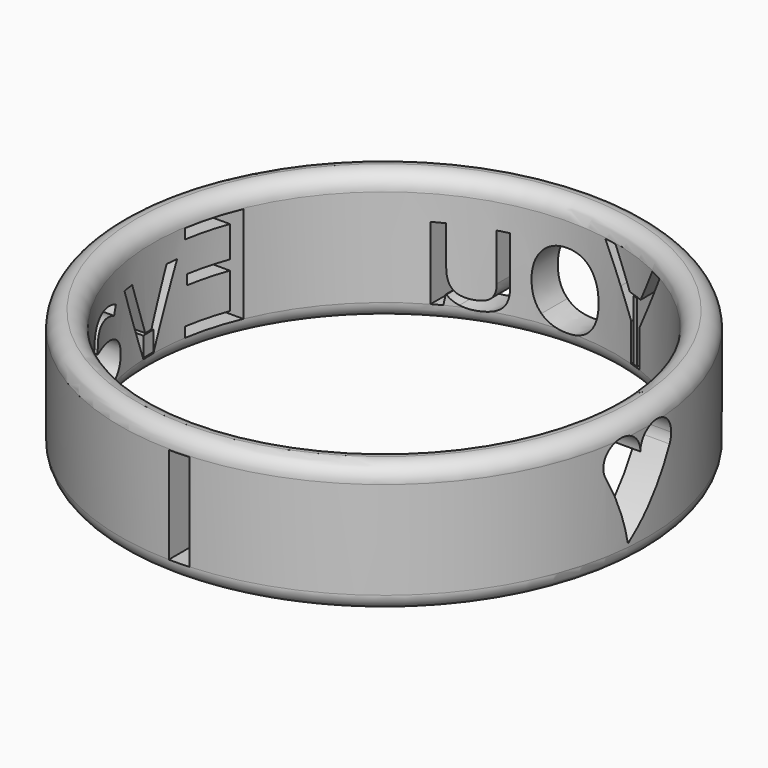
from build123d import *

# Parameters (mm, degrees)
F0_R          = 32.5
F0_R_2        = 28.5
F1_DEPTH      = 16
F3_TEXT_SIZE  = 16.6666666667
F4_DEPTH      = 25
F7_DEPTH      = 25
F15_TEXT_SIZE = 16.6666666667
F16_DEPTH     = 25
F17_DEPTH     = 25
F19_DEPTH     = 1.5
F19_TAPER     = -45
F21_DEPTH     = 2.7213541667
F22_DEPTH     = 0.15
F23_DEPTH     = 0.15
F24_DEPTH     = 7.6968030557
F25_DEPTH     = 0.15
F26_DEPTH     = 0.15
F24_FACE2_W   = 4.1758402468
F24_FACE2_H   = 7.3968030557
F27_DEPTH     = 0.4
F27_TAPER     = -45
F24_FACE3_W   = 4.2422939469
F24_FACE3_H   = 7.3968030557
F28_DEPTH     = 0.4
F28_TAPER     = -45


# Not quite as in the source:
# - a fillet or chamfer that OpenCascade refuses, or shapes differently, is made with other operations: its cross-section is extruded or revolved along the edge and cut away or added
# - Text() gives the source's letters only with a copy of the font that has no kerning and outlines rounded to 1/6400 em; it was checked with that copy


with BuildPart() as f1:
    # F0 (on Top) → F1 (new body)
    with BuildSketch(Plane.XY):
        Circle(F0_R)
        Circle(F0_R_2, mode=Mode.SUBTRACT)
    extrude(amount=F1_DEPTH)

    # F3 (on offset) → F4 (cut)
    with BuildSketch(Plane.XZ.offset(36)):
        with Locations((-2.0104166667, 2)):
            Text('I', F3_TEXT_SIZE, font='Open Sans', font_style=FontStyle.BOLD, text_align=(TextAlign.LEFT, TextAlign.BOTTOM))
    extrude(amount=-F4_DEPTH, mode=Mode.SUBTRACT)

    # F6 (on offset) → F7 (cut)
    with BuildSketch(Plane.YZ.offset(35.5)):
        with BuildLine():
            ThreePointArc((3.57761604, 10.5411187726), (0.7657574334, 9.2722506178), (-1.1375576102, 11.7))
            ThreePointArc((-1.1375576102, 11.7), (-3.0145179727, 9.2788800918), (-5.8270148983, 10.493237064))
            ThreePointArc((-5.8270148983, 10.493237064), (-4.0497196394, 6.5648465547), (-2.9116181205, 2.4060299726))
            ThreePointArc((-2.9116181205, 2.4060299726), (0.7233061967, 6.1622323434), (3.57761604, 10.5411187726))
        make_face()
        with BuildLine():
            ThreePointArc((-5.8270148983, 10.493237064), (-3.0145179727, 9.2788800918), (-1.1375576102, 11.7))
            ThreePointArc((-1.1375576102, 11.7), (-4.2605972477, 14.1211199082), (-5.8270148983, 10.493237064))
        make_face()
        with BuildLine():
            ThreePointArc((3.8624423898, 11.7), (1.3624423898, 14.2), (-1.1375576102, 11.7))
            ThreePointArc((-1.1375576102, 11.7), (0.7657574334, 9.2722506178), (3.57761604, 10.5411187726))
            ThreePointArc((3.57761604, 10.5411187726), (3.790191772, 11.1033150436), (3.8624423898, 11.7))
        make_face()
    extrude(amount=-F7_DEPTH, mode=Mode.SUBTRACT)

    # F15 (on line) → F16 (cut)
    with BuildSketch(Plane(origin=(-35.5, 0, 0), x_dir=(0, -1, 0), z_dir=(-1, 0, 0))):
        with Locations((-12.7682291667, 2)):
            Text('Eva', F15_TEXT_SIZE, font='Open Sans', text_align=(TextAlign.LEFT, TextAlign.BOTTOM))
        with BuildLine():
            add(Edge.make_bspline(
                [(7.4739583333, 3.3346354167), (7.9166666667, 2.953125), (8.7135416667, 2.953125)],
                knots=[0, 0, 0, 1, 1, 1], degree=2))
            add(Edge.make_bspline(
                [(8.7135416667, 2.953125), (9.9765625, 2.953125), (10.6966145833, 3.64453125)],
                knots=[0, 0, 0, 1, 1, 1], degree=2))
            add(Edge.make_bspline(
                [(10.6966145833, 3.64453125), (11.4166666667, 4.3359375), (11.4166666667, 5.5807291667)],
                knots=[0, 0, 0, 1, 1, 1], degree=2))
            Line((11.4166666667, 5.5807291667), (11.4166666667, 6.3854166667))
            Line((11.4166666667, 6.3854166667), (10.0651041667, 6.3307291667))
            add(Edge.make_bspline(
                [(10.0651041667, 6.3307291667), (8.453125, 6.2734375), (7.7421875, 5.8294270833)],
                knots=[0, 0, 0, 1, 1, 1], degree=2))
            add(Edge.make_bspline(
                [(7.7421875, 5.8294270833), (7.03125, 5.3854166667), (7.03125, 4.4505208333)],
                knots=[0, 0, 0, 1, 1, 1], degree=2))
            add(Edge.make_bspline(
                [(7.03125, 4.4505208333), (7.03125, 3.7161458333), (7.4739583333, 3.3346354167)],
                knots=[0, 0, 0, 1, 1, 1], degree=2))
        make_face()
    extrude(amount=-F16_DEPTH, mode=Mode.SUBTRACT)

    # F11 (on line) → F17 (cut)
    with BuildSketch(Plane(origin=(0, 35.5, 0), x_dir=(-1, 0, 0), z_dir=(0, 1, 0))):
        Polygon((-14.0989583333, 13.8984375), (-11.8328748379, 9.6968030557), (-10.3610019737, 9.6968030557), (-12.5859375, 13.8984375), align=None)
        Polygon((-10.3610019737, 9.6968030557), (-11.8328748379, 9.6968030557), (-10.1354166667, 6.5494791667), (-10.1354166667, 2), (-8.7369791667, 2), (-8.7369791667, 6.6145833333), (-7.0564696648, 9.6968030557), (-8.5026666772, 9.6968030557), (-9.4348958333, 7.9479166667), align=None)
        Polygon((-8.5026666772, 9.6968030557), (-10.3610019737, 9.6968030557), (-9.4348958333, 7.9479166667), align=None)
        Polygon((-6.2630208333, 13.8984375), (-8.5026666772, 9.6968030557), (-7.0564696648, 9.6968030557), (-4.765625, 13.8984375), align=None)
        with BuildLine():
            add(Edge.make_bspline(
                [(4.3645833333, 6.46875), (4.3645833333, 4.2864583333), (3.2669270833, 3.0611979167)],
                knots=[0, 0, 0, 1, 1, 1], degree=2))
            add(Edge.make_bspline(
                [(3.26171875, 9.8372395833), (4.3645833333, 8.5911458333), (4.3645833333, 6.46875)],
                knots=[0, 0, 0, 1, 1, 1], degree=2))
            add(Edge.make_bspline(
                [(0.2890625, 11.0833333333), (2.1588541667, 11.0833333333), (3.26171875, 9.8372395833)],
                knots=[0, 0, 0, 1, 1, 1], degree=2))
            add(Edge.make_bspline(
                [(-2.7395833333, 9.8658854167), (-1.6484375, 11.0833333333), (0.2890625, 11.0833333333)],
                knots=[0, 0, 0, 1, 1, 1], degree=2))
            add(Edge.make_bspline(
                [(-3.8307291667, 6.46875), (-3.8307291667, 8.6484375), (-2.7395833333, 9.8658854167)],
                knots=[0, 0, 0, 1, 1, 1], degree=2))
            add(Edge.make_bspline(
                [(-3.3255208333, 4.0104166667), (-3.8307291667, 5.0598958333), (-3.8307291667, 6.46875)],
                knots=[0, 0, 0, 1, 1, 1], degree=2))
            add(Edge.make_bspline(
                [(-1.8932291667, 2.3984375), (-2.8203125, 2.9609375), (-3.3255208333, 4.0104166667)],
                knots=[0, 0, 0, 1, 1, 1], degree=2))
            add(Edge.make_bspline(
                [(0.2317708333, 1.8359375), (-0.9661458333, 1.8359375), (-1.8932291667, 2.3984375)],
                knots=[0, 0, 0, 1, 1, 1], degree=2))
            add(Edge.make_bspline(
                [(3.2669270833, 3.0611979167), (2.1692708333, 1.8359375), (0.2317708333, 1.8359375)],
                knots=[0, 0, 0, 1, 1, 1], degree=2))
        make_face()
        with BuildLine():
            add(Edge.make_bspline(
                [(-2.4296875, 6.46875), (-2.4296875, 4.7578125), (-1.74609375, 3.86328125)],
                knots=[0, 0, 0, 1, 1, 1], degree=2))
            add(Edge.make_bspline(
                [(-1.75390625, 9.0638020833), (-2.4296875, 8.1927083333), (-2.4296875, 6.46875)],
                knots=[0, 0, 0, 1, 1, 1], degree=2))
            add(Edge.make_bspline(
                [(0.2473958333, 9.9348958333), (-1.078125, 9.9348958333), (-1.75390625, 9.0638020833)],
                knots=[0, 0, 0, 1, 1, 1], degree=2))
            add(Edge.make_bspline(
                [(2.2786458333, 9.0520833333), (1.5911458333, 9.9348958333), (0.2473958333, 9.9348958333)],
                knots=[0, 0, 0, 1, 1, 1], degree=2))
            add(Edge.make_bspline(
                [(2.9661458333, 6.46875), (2.9661458333, 8.1692708333), (2.2786458333, 9.0520833333)],
                knots=[0, 0, 0, 1, 1, 1], degree=2))
            add(Edge.make_bspline(
                [(2.2786458333, 3.859375), (2.9661458333, 4.75), (2.9661458333, 6.46875)],
                knots=[0, 0, 0, 1, 1, 1], degree=2))
            add(Edge.make_bspline(
                [(0.2630208333, 2.96875), (1.5911458333, 2.96875), (2.2786458333, 3.859375)],
                knots=[0, 0, 0, 1, 1, 1], degree=2))
            add(Edge.make_bspline(
                [(-1.74609375, 3.86328125), (-1.0625, 2.96875), (0.2630208333, 2.96875)],
                knots=[0, 0, 0, 1, 1, 1], degree=2))
        make_face(mode=Mode.SUBTRACT)
        with BuildLine():
            Line((8.0052083333, 5.1328125), (8.0052083333, 10.9192708333))
            Line((8.0052083333, 10.9192708333), (6.6380208333, 10.9192708333))
            Line((6.6380208333, 10.9192708333), (6.6380208333, 5.0833333333))
            add(Edge.make_bspline(
                [(7.4466145833, 2.609375), (6.6380208333, 3.3828125), (6.6380208333, 5.0833333333)],
                knots=[0, 0, 0, 1, 1, 1], degree=2))
            add(Edge.make_bspline(
                [(9.8828125, 1.8359375), (8.2552083333, 1.8359375), (7.4466145833, 2.609375)],
                knots=[0, 0, 0, 1, 1, 1], degree=2))
            add(Edge.make_bspline(
                [(11.5651041667, 2.1861979167), (10.828125, 1.8359375), (9.8828125, 1.8359375)],
                knots=[0, 0, 0, 1, 1, 1], degree=2))
            add(Edge.make_bspline(
                [(12.7161458333, 3.1953125), (12.3020833333, 2.5364583333), (11.5651041667, 2.1861979167)],
                knots=[0, 0, 0, 1, 1, 1], degree=2))
            Line((12.7161458333, 3.1953125), (12.7890625, 3.1953125))
            Line((12.7890625, 3.1953125), (12.984375, 2))
            Line((12.984375, 2), (14.0989583333, 2))
            Line((14.0989583333, 2), (14.0989583333, 10.9192708333))
            Line((14.0989583333, 10.9192708333), (12.7473958333, 10.9192708333))
            Line((12.7473958333, 10.9192708333), (12.7473958333, 6.2317708333))
            add(Edge.make_bspline(
                [(12.1015625, 3.7330729167), (12.7473958333, 4.4973958333), (12.7473958333, 6.2317708333)],
                knots=[0, 0, 0, 1, 1, 1], degree=2))
            add(Edge.make_bspline(
                [(10.0546875, 2.96875), (11.4557291667, 2.96875), (12.1015625, 3.7330729167)],
                knots=[0, 0, 0, 1, 1, 1], degree=2))
            add(Edge.make_bspline(
                [(8.5013020833, 3.5052083333), (8.9973958333, 2.96875), (10.0546875, 2.96875)],
                knots=[0, 0, 0, 1, 1, 1], degree=2))
            add(Edge.make_bspline(
                [(8.0052083333, 5.1328125), (8.0052083333, 4.0416666667), (8.5013020833, 3.5052083333)],
                knots=[0, 0, 0, 1, 1, 1], degree=2))
        make_face()
        with BuildLine():
            add(Edge.make_bspline(
                [(-1.75390625, 9.0638020833), (-2.4296875, 8.1927083333), (-2.4296875, 6.46875)],
                knots=[0, 0, 0, 1, 1, 1], degree=2))
            add(Edge.make_bspline(
                [(-2.4296875, 6.46875), (-2.4296875, 4.7578125), (-1.74609375, 3.86328125)],
                knots=[0, 0, 0, 1, 1, 1], degree=2))
            add(Edge.make_bspline(
                [(-1.74609375, 3.86328125), (-1.0625, 2.96875), (0.2630208333, 2.96875)],
                knots=[0, 0, 0, 1, 1, 1], degree=2))
            add(Edge.make_bspline(
                [(0.2630208333, 2.96875), (1.5911458333, 2.96875), (2.2786458333, 3.859375)],
                knots=[0, 0, 0, 1, 1, 1], degree=2))
            add(Edge.make_bspline(
                [(2.2786458333, 3.859375), (2.9661458333, 4.75), (2.9661458333, 6.46875)],
                knots=[0, 0, 0, 1, 1, 1], degree=2))
            add(Edge.make_bspline(
                [(2.9661458333, 6.46875), (2.9661458333, 8.1692708333), (2.2786458333, 9.0520833333)],
                knots=[0, 0, 0, 1, 1, 1], degree=2))
            add(Edge.make_bspline(
                [(2.2786458333, 9.0520833333), (1.5911458333, 9.9348958333), (0.2473958333, 9.9348958333)],
                knots=[0, 0, 0, 1, 1, 1], degree=2))
            add(Edge.make_bspline(
                [(0.2473958333, 9.9348958333), (-1.078125, 9.9348958333), (-1.75390625, 9.0638020833)],
                knots=[0, 0, 0, 1, 1, 1], degree=2))
        make_face()
    extrude(amount=-F17_DEPTH, mode=Mode.SUBTRACT)

    # F18: fillet of radius 2 on 4 edges, made by hand

    # F18_s1 → F18_t2 (revolve, cut)
    with BuildSketch(Plane.XZ):
        with BuildLine():
            ThreePointArc((32.5, 14), (31.9142135624, 15.4142135624), (30.5, 16))
            Line((30.5, 16), (32.5, 16))
            Line((32.5, 16), (32.5, 14))
        make_face()
    revolve(axis=Axis((0, 0, 16), (0, 0, 1)), mode=Mode.SUBTRACT)

    # F18_s3 → F18_t4 (revolve, cut)
    with BuildSketch(Plane.XZ):
        with BuildLine():
            ThreePointArc((30.5, 16), (29.0857864376, 15.4142135624), (28.5, 14))
            Line((28.5, 14), (28.5, 16))
            Line((28.5, 16), (30.5, 16))
        make_face()
    revolve(axis=Axis((0, 0, 16), (0, 0, 1)), mode=Mode.SUBTRACT)

    # F18_s5 → F18_t6 (revolve, cut)
    with BuildSketch(Plane.XZ):
        with BuildLine():
            ThreePointArc((32.5, 2), (31.9142135624, 0.5857864376), (30.5, 0))
            Line((30.5, 0), (32.5, 0))
            Line((32.5, 0), (32.5, 2))
        make_face()
    revolve(axis=Axis((0, 0, 0), (0, 0, 1)), mode=Mode.SUBTRACT)

    # F18_s7 → F18_t8 (revolve, cut)
    with BuildSketch(Plane.XZ):
        with BuildLine():
            ThreePointArc((30.5, 0), (29.0857864376, 0.5857864376), (28.5, 2))
            Line((28.5, 2), (28.5, 0))
            Line((28.5, 0), (30.5, 0))
        make_face()
    revolve(axis=Axis((0, 0, 0), (0, 0, 1)), mode=Mode.SUBTRACT)

    # F16_face (on face) → F19 (cut)
    with BuildSketch(Plane(origin=(-30.492647224, -0.6679690048, 3.2213541667), x_dir=(1, 0, 0), z_dir=(0, 0, -1))):
        with BuildLine():
            ThreePointArc((-1.9998022152, 0.0325518285), (-2.0004877017, 8.04e-08), (-2.001140577, -0.0325523382))
            Line((-2.001140577, -0.0325523382), (1.999731514, -0.0325523382))
            ThreePointArc((1.999731514, -0.0325523382), (2.0004760683, 1.811e-07), (2.0012578131, 0.0325518285))
            Line((2.0012578131, 0.0325518285), (-1.9998022152, 0.0325518285))
        make_face()
    extrude(amount=-F19_DEPTH, taper=F19_TAPER, mode=Mode.SUBTRACT)


with BuildPart() as f21:
    # F20 (on face) → F21 (new body, through all)
    with BuildSketch(Plane.XY.offset(2)):
        with BuildLine():
            Line((-28.4997696598, 0.1145833333), (-32.4997980095, 0.1145833333))
            ThreePointArc((-32.4997980095, 0.1145833333), (-32.4929963134, -0.6746781304), (-32.467030135, -1.4635416667))
            Line((-32.467030135, -1.4635416667), (-28.4623970493, -1.4635416667))
            ThreePointArc((-28.4623970493, -1.4635416667), (-28.4920116642, -0.6747379671), (-28.4997696598, 0.1145833333))
        make_face()
    extrude(amount=F21_DEPTH)

    # F22 (cut): a face of the model
    f22_faces = [f21.faces().sort_by_distance(p)[0] for p in [
        (-30.4890855492, -0.6746304437, 4.7213541667),
    ]]
    extrude(f22_faces, amount=-F22_DEPTH, mode=Mode.SUBTRACT)

    # F23 (cut): a face of the model
    f23_faces = [f21.faces().sort_by_distance(p)[0] for p in [
        (-30.4890855492, -0.6746304437, 2),
    ]]
    extrude(f23_faces, amount=-F23_DEPTH, mode=Mode.SUBTRACT)


with BuildPart() as f24:
    # F24 (new, through all): a face of the model
    f24_faces = [f1.part.faces().sort_by_distance(p)[0] for p in [
        (9.4380375274, 28.9925153883, 2),
    ]]
    extrude(f24_faces, amount=F24_DEPTH)

    # F25 (cut): a face of the model
    f25_faces = [f24.faces().sort_by_distance(p)[0] for p in [
        (9.4380375274, 28.9925153883, 9.6968030557),
    ]]
    extrude(f25_faces, amount=-F25_DEPTH, mode=Mode.SUBTRACT)

    # F26 (cut): a face of the model
    f26_faces = [f24.faces().sort_by_distance(p)[0] for p in [
        (9.4380375274, 28.9925153883, 2),
    ]]
    extrude(f26_faces, amount=-F26_DEPTH, mode=Mode.SUBTRACT)

    # F24_face2 (on face) → F27 (cut)
    with BuildSketch(Plane(origin=(8.7369791667, 29.2156770348, 5.8484015279), x_dir=(0, -1, 0), z_dir=(-1, 0, 0))):
        Rectangle(F24_FACE2_W, F24_FACE2_H)
    extrude(amount=-F27_DEPTH, taper=F27_TAPER, mode=Mode.SUBTRACT)

    # F24_face3 (on face) → F28 (cut)
    with BuildSketch(Plane(origin=(10.1354166667, 28.7580260886, 5.8484015279), x_dir=(0, 1, 0), z_dir=(1, 0, 0))):
        Rectangle(F24_FACE3_W, F24_FACE3_H)
    extrude(amount=-F28_DEPTH, taper=F28_TAPER, mode=Mode.SUBTRACT)


solid = Compound([f1.part, f21.part, f24.part])
